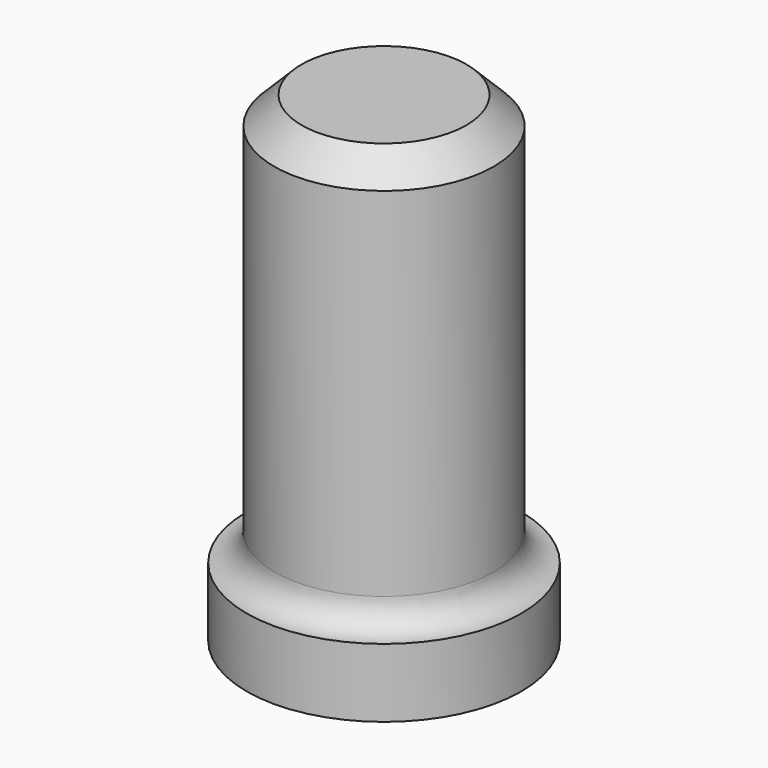
from build123d import *

# Parameters (mm, degrees)
F0_W    = 6
F0_H    = 22.5
F2_SIZE = 1.5
F3_R    = 1.49999


# Not quite as in the source:
# - a fillet or chamfer is up to 0.001 mm smaller than in the source, because OpenCascade refuses the exact size


with BuildPart() as f1:
    # F0 (on Front) → F1 (revolve)
    with BuildSketch(Plane.XZ):
        with Locations((3, 11.25)):
            Rectangle(F0_W, F0_H)
        Polygon((6, 0), (0, 0), (0, -3.75), (7.5, -3.75), (7.5, 0), align=None)
    revolve(axis=Axis((0, 0, 8.5798527999), (0, 0, -1)))

    # F2
    f2_edges = [f1.edges().sort_by_distance(p)[0] for p in [
        (-6, 0, 22.5),
    ]]
    chamfer(f2_edges, length=F2_SIZE)

    # F3 (radius 1.5 in the source; OpenCascade refuses exactly that, so slightly less here)
    f3_edges = [f1.edges().sort_by_distance(p)[0] for p in [
        (-6, 0, 0),
    ]]
    fillet(f3_edges, radius=F3_R)


solid = f1.part
